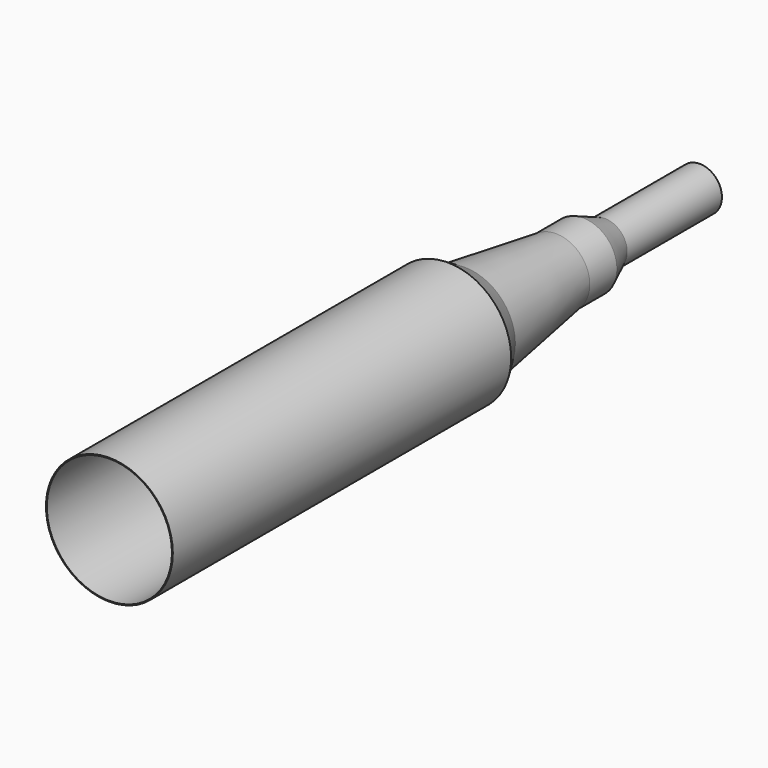
from build123d import *

# Parameters (mm, degrees)
F0_R         = 15
F1_DEPTH     = 100
F1_FACE_R    = 15
F3_R         = 12
F6_R         = 8
F4_FACE_R    = 12
F8_DEPTH     = 8
F8_FACE_R    = 8
F10_R        = 5.25
F12_DEPTH    = 28
F13_T        = 0.2
F13_T4_ANGLE = 180.000000001
F13_T6_ANGLE = 180.000000001


# Not quite as in the source:
# - a shell that OpenCascade refuses in one call is made with other operations: the cavity is built on its own and cut out


with BuildPart() as f1:
    # F0 (on Front) → F1 (new body)
    with BuildSketch(Plane.XZ):
        Circle(F0_R)
    extrude(amount=-F1_DEPTH)

    # F1_face (on face) → F4 section 0
    with BuildSketch(Plane(origin=(0, 100, 0), x_dir=(1, 0, 0), z_dir=(0, 1, 0))):
        Circle(F1_FACE_R)
    # F3 (on offset) → F4 section 1
    with BuildSketch(Plane(origin=(0, 105, 0), x_dir=(-1, 0, 0), z_dir=(0, 1, 0))):
        Circle(F3_R)
    loft()

    # F6 (on offset) → F7 section 0
    with BuildSketch(Plane(origin=(0, 132, 0), x_dir=(-1, 0, 0), z_dir=(0, 1, 0))):
        Circle(F6_R)
    # F4_face (on face) → F7 section 1
    with BuildSketch(Plane(origin=(0, 105, 0), x_dir=(-1, 0, 0), z_dir=(0, 1, 0))):
        Circle(F4_FACE_R)
    loft()

    # F8 (add): a face of the model
    f8_faces = [f1.faces().sort_by_distance(p)[0] for p in [
        (0, 132, 0),
    ]]
    extrude(f8_faces, amount=F8_DEPTH)

    # F8_face (on face) → F11 section 0
    with BuildSketch(Plane(origin=(0, 140, 0), x_dir=(-1, 0, 0), z_dir=(0, 1, 0))):
        Circle(F8_FACE_R)
    # F10 (on offset) → F11 section 1
    with BuildSketch(Plane(origin=(0, 146.5, 0), x_dir=(-1, 0, 0), z_dir=(0, 1, 0))):
        Circle(F10_R)
    loft()

    # F12 (add): a face of the model
    f12_faces = [f1.faces().sort_by_distance(p)[0] for p in [
        (0, 146.5, 0),
    ]]
    extrude(f12_faces, amount=F12_DEPTH)

    # F13: shell of thickness 0.2, made by hand


with BuildPart() as f13_core1:
    # F13_t2: copy of F1
    add(f1.part)

    # the walls: a layer under each face that stays
    f13_faces = [f13_core1.faces().sort_by_distance(p)[0] for p in [
        (-15, 50, 0),
        (-13.5, 102.5, 0),
        (10, 118.5, 0),
        (8, 136, 0),
        (6.625, 143.25, 0),
        (5.25, 160.5, 0),
    ]]
    thicken(f13_faces, amount=-F13_T, mode=Mode.SUBTRACT)

    # F13_s3 → F13_t4 (revolve, cut)
    with BuildSketch(Plane.XY):
        Polygon((-12.0036933928, 105.0013220888), (-11.8285014149, 104.8971008489), (-11.807999158, 104.931271277), (-11.8021593075, 104.9706902678), align=None)
    revolve(axis=Axis((0, 105, 0), (0, -1, 0)), revolution_arc=F13_T4_ANGLE, mode=Mode.SUBTRACT)

    # F13_s5 → F13_t6 (revolve, cut)
    with BuildSketch(Plane.XY):
        Polygon((12.0036933928, 105.0013220888), (11.8285014149, 104.8971008489), (11.807999158, 104.931271277), (11.8021593075, 104.9706902678), align=None)
    revolve(axis=Axis((0, 105, 0), (0, -1, 0)), revolution_arc=F13_T6_ANGLE, mode=Mode.SUBTRACT)

    # F13_s7 → F13_t8 (revolve, cut)
    with BuildSketch(Plane.XY):
        Polygon((-8.0039784069, 132.0002930973), (-7.8021593075, 131.9706902678), (-7.8, 131.9852655936), (-7.8, 132), align=None)
    revolve(axis=Axis((0, 132, 0), (0, 1, 0)), mode=Mode.SUBTRACT)

    # F13_s9 → F13_t10 (revolve, cut)
    with BuildSketch(Plane.XY):
        Polygon((-5.2538419345, 146.50077928), (-5.0658065498, 146.4220720018), (-5.05, 146.4594329377), (-5.05, 146.5), align=None)
    revolve(axis=Axis((0, 146.5, 0), (0, 1, 0)), mode=Mode.SUBTRACT)


with BuildPart() as f1_1:
    add(f1.part)

    # what is left inside the walls is the cavity
    f13_cavity = [f13_core1.part.solids().sort_by_distance(p)[0] for p in [
        (-14.798, 66.629735, 0),
    ]]
    add(f13_cavity, mode=Mode.SUBTRACT)


solid = f1_1.part
